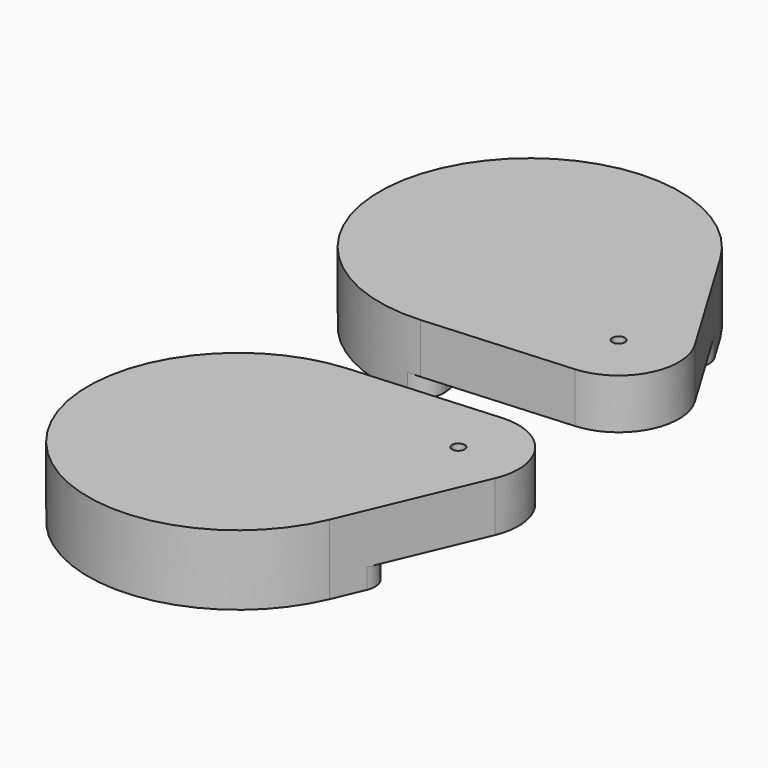
from build123d import *

# Parameters (mm, degrees)
F1_DEPTH    = 8.89
F2_W        = 52.2928647697
F2_H        = 32.6345004141
F3_DEPTH    = 2.54
F4_R        = 3.175
F5_DEPTH    = 2.54
F6_R        = 0.79375
F7_DEPTH    = 6.351
F8_T1_DEPTH = 7.4013341754
F8_T3_DEPTH = 12.1194356419
F8_T5_DEPTH = 9.8986940254


# Not quite as in the source:
# - a fillet or chamfer that OpenCascade refuses, or shapes differently, is made with other operations: its cross-section is extruded or revolved along the edge and cut away or added


with BuildPart() as f1:
    # F0 (on Top) → F1 (new body)
    with BuildSketch(Plane.XY):
        with BuildLine():
            Line((17.2489482218, 20.3014724895), (-1.3276294456, 19.0036812238))
            ThreePointArc((-1.3276294456, 19.0036812238), (-15.5016226265, -11.0725875903), (17.5458726888, -7.4192217643))
            Line((17.5458726888, -7.4192217643), (24.7983490755, 9.7323112943))
            ThreePointArc((24.7983490755, 9.7323112943), (23.9806490506, 17.1290350361), (17.2489482218, 20.3014724895))
        make_face()
    extrude(amount=F1_DEPTH)

    # F2 (on face) → F3 (cut)
    with BuildSketch(Plane(origin=(0, 0, 0), x_dir=(1, 0, 0), z_dir=(0, 0, -1))):
        with Locations((26.1464323848, -16.3172502071)):
            Rectangle(F2_W, F2_H)
    extrude(amount=-F3_DEPTH, mode=Mode.SUBTRACT)

    # F4 (on face) → F5 (cut, through all)
    with BuildSketch(Plane(origin=(0, 0, 0), x_dir=(1, 0, 0), z_dir=(0, 0, -1))):
        Circle(F4_R)
    extrude(amount=-F5_DEPTH, mode=Mode.SUBTRACT)

    # F6 (on face) → F7 (cut, through all)
    with BuildSketch(Plane(origin=(0, 0, 2.54), x_dir=(1, 0, 0), z_dir=(0, 0, -1))):
        with Locations((17.78, -12.7)):
            Circle(F6_R)
    extrude(amount=-F7_DEPTH, mode=Mode.SUBTRACT)

    # F8: fillet of radius 2.54 on 4 edges, made by hand

    # F8_s2 → F8_t1 (cut)
    with BuildSketch(Plane.XY.offset(-4.8613341754)):
        with BuildLine():
            ThreePointArc((5.1195336702, 0), (3.7808361274, -0.3814150726), (2.8441853723, -1.4111111111))
            ThreePointArc((2.8441853723, -1.4111111111), (3.091190188, -0.7246849118), (3.175, 0))
            Line((3.175, 0), (5.1195336702, 0))
        make_face()
        with BuildLine():
            ThreePointArc((0, 5.1195336702), (-0.3814150726, 3.7808361274), (-1.4111111111, 2.8441853723))
            ThreePointArc((-1.4111111111, 2.8441853723), (-0.7246849118, 3.091190188), (0, 3.175))
            Line((0, 3.175), (0, 5.1195336702))
        make_face()
    extrude(amount=F8_T1_DEPTH, mode=Mode.SUBTRACT)

    # F8_s4 → F8_t3 (cut)
    with BuildSketch(Plane.XY.offset(-9.5794356419)):
        with BuildLine():
            ThreePointArc((19.1907446922, -3.5292295686), (18.9683971595, -1.1366189228), (16.8512950004, 0))
            Line((16.8512950004, 0), (20.6830692572, 0))
            Line((20.6830692572, 0), (19.1907446922, -3.5292295686))
        make_face()
    extrude(amount=F8_T3_DEPTH, mode=Mode.SUBTRACT)

    # F8_s6 → F8_t5 (cut)
    with BuildSketch(Plane.XY.offset(-7.3586940254)):
        with BuildLine():
            ThreePointArc((-2.9307692308, 18.8232062018), (-0.8878731656, 18.2427138692), (0, 16.3134453749))
            Line((0, 16.3134453749), (0.254, 16.3134453749))
            Line((0.254, 16.3134453749), (0.254, 19.0964316717))
            Line((0.254, 19.0964316717), (-0.0177017259, 19.349814088))
            ThreePointArc((-0.0177017259, 19.349814088), (-1.3453311715, 19.2570636401), (-2.9698461538, 19.0741822845))
            Line((-2.9698461538, 19.0741822845), (-2.9307692308, 18.8232062018))
        make_face()
    extrude(amount=F8_T5_DEPTH, mode=Mode.SUBTRACT)


with BuildPart() as f10_1:
    # F10: instance of F1
    add(f1.part.mirror(Plane(origin=(7.5181162396, 25.9871372646, 5.715), x_dir=(-0.9975685682, -0.0696918344, 0), z_dir=(-0.0696918344, 0.9975685682, 0))))


solid = Compound([f1.part, f10_1.part])
